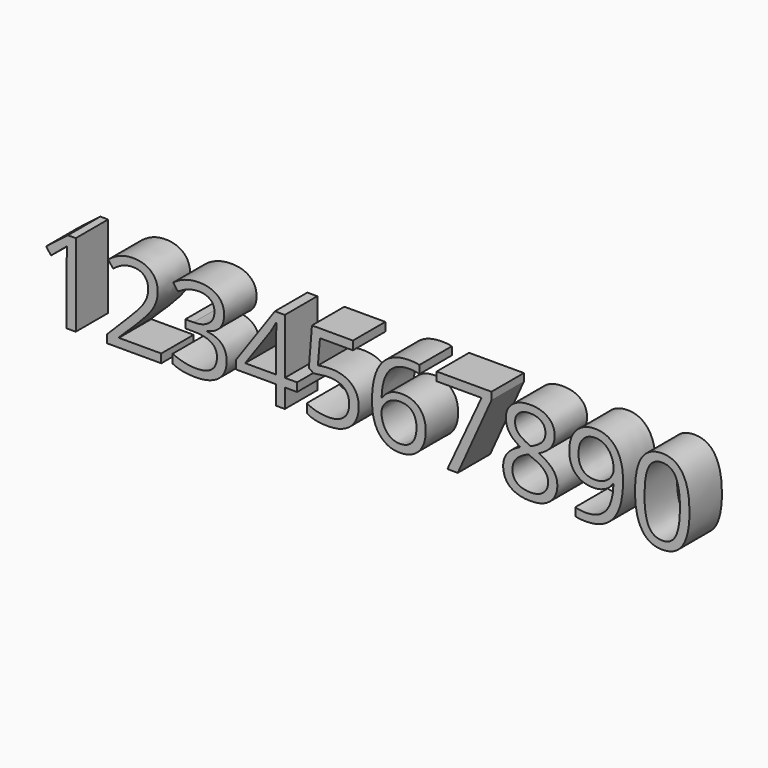
from build123d import *

# Parameters (mm, degrees)
F0_TEXT_SIZE = 71.2234837313
F1_DEPTH     = 25


# Not quite as in the source:
# - Text() gives the source's letters only with a copy of the font that has no kerning and outlines rounded to 1/6400 em; it was checked with that copy


with BuildPart() as f1:
    # F0 (on Front) → F1 (new body)
    with BuildSketch(Plane.XZ):
        with Locations((-149.3840515614, -88.5410010815)):
            Text('1234567890', F0_TEXT_SIZE, font='Open Sans', text_align=(TextAlign.LEFT, TextAlign.BOTTOM))
    extrude(amount=F1_DEPTH)


solid = f1.part
